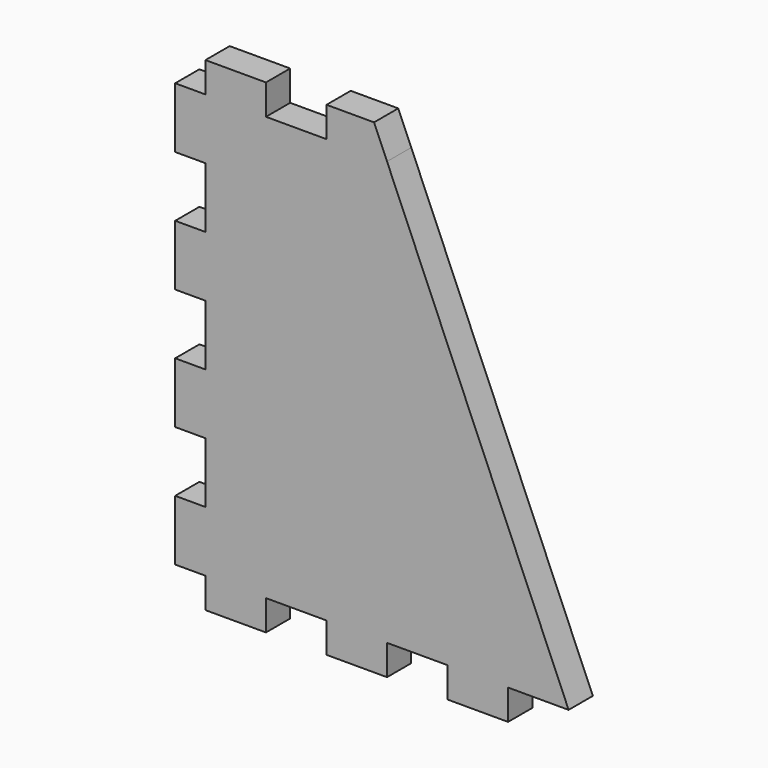
from build123d import *

# Parameters (mm, degrees)
F1_DEPTH = 10


# Not quite as in the source:
# - a feature names something its author has since deleted; it is built from what else it names


with BuildPart() as f1:
    # F0 (on Front) → F1 (new body)
    with BuildSketch(Plane.XZ):
        Polygon((260, -100), (260, -110), (280, -110), (280, -100), (300, -100), (300, -110), (320, -110), (320, -100), (340, -100), (340, -110), (360, -110), (360, -100), (380, -100), (320, 40), (315.7142857143, 50), (300, 50), (300, 40), (280, 40), (280, 50), (260, 50), (260, 40), (250, 40), (250, 20), (260, 20), (260, 0), (250, 0), (250, -20), (260, -20), (260, -40), (250, -40), (250, -60), (260, -60), (260, -80), (250, -80), (250, -100), align=None)
    extrude(amount=-F1_DEPTH)


solid = f1.part
